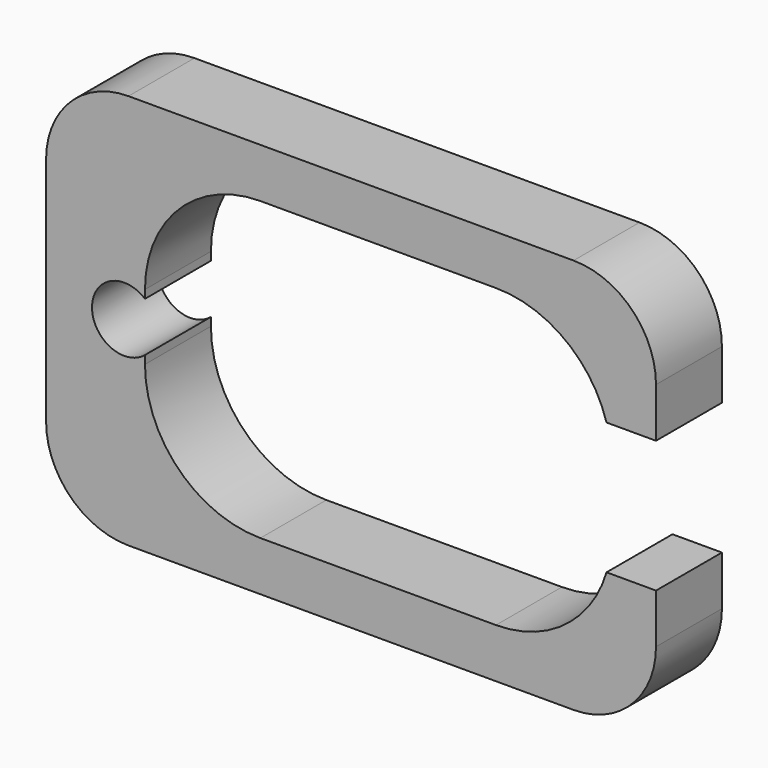
from build123d import *

# Parameters (mm, degrees)
F1_DEPTH    = 2.5
F2_R        = 5
F3_T1_DEPTH = 5


# Not quite as in the source:
# - a fillet or chamfer that OpenCascade refuses, or shapes differently, is made with other operations: its cross-section is extruded or revolved along the edge and cut away or added


with BuildPart() as f1:
    # F0 (on Front) → F1 (new body, symmetric)
    with BuildSketch(Plane.XZ):
        with BuildLine():
            Line((18.5, 12), (-18.5, 12))
            Line((-18.5, 12), (-18.5, -12))
            Line((-18.5, -12), (18.5, -12))
            Line((18.5, -12), (18.5, -4))
            Line((18.5, -4), (15.5, -4))
            Line((15.5, -4), (15.5, -9))
            Line((15.5, -9), (-12.5, -9))
            Line((-12.5, -9), (-12.5, -1.5))
            ThreePointArc((-12.5, -1.5), (-15.714868952, 0), (-12.5, 1.5))
            Line((-12.5, 1.5), (-12.5, 9))
            Line((-12.5, 9), (15.5, 9))
            Line((15.5, 9), (15.5, 4))
            Line((15.5, 4), (18.5, 4))
            Line((18.5, 4), (18.5, 12))
        make_face()
    extrude(amount=F1_DEPTH, both=True)

    # F2
    f2_edges = [f1.edges().sort_by_distance(p)[0] for p in [
        (-18.5, 0, 12),
        (18.5, 0, 12),
        (18.5, 0, -12),
        (-18.5, 0, -12),
    ]]
    fillet(f2_edges, radius=F2_R)

    # F3: fillet of radius 7 on 4 edges, made by hand

    # F3_s2 → F3_t1 (join)
    with BuildSketch(Plane.XZ.offset(-2.5)):
        with BuildLine():
            ThreePointArc((15.5, 4), (12.9750962002, 7.6124860802), (8.7917960675, 9))
            Line((8.7917960675, 9), (15.5, 9))
            Line((15.5, 9), (15.5, 4))
        make_face()
        with BuildLine():
            ThreePointArc((15.5, -4), (12.9750962002, -7.6124860802), (8.7917960675, -9))
            Line((8.7917960675, -9), (15.5, -9))
            Line((15.5, -9), (15.5, -4))
        make_face()
        with BuildLine():
            ThreePointArc((-12.5, -2), (-10.4497474683, -6.9497474683), (-5.5, -9))
            Line((-5.5, -9), (-12.5, -9))
            Line((-12.5, -9), (-12.5, -2))
        make_face()
        with BuildLine():
            ThreePointArc((-5.5, 9), (-10.4497474683, 6.9497474683), (-12.5, 2))
            Line((-12.5, 2), (-12.5, 9))
            Line((-12.5, 9), (-5.5, 9))
        make_face()
    extrude(amount=F3_T1_DEPTH)


solid = f1.part
